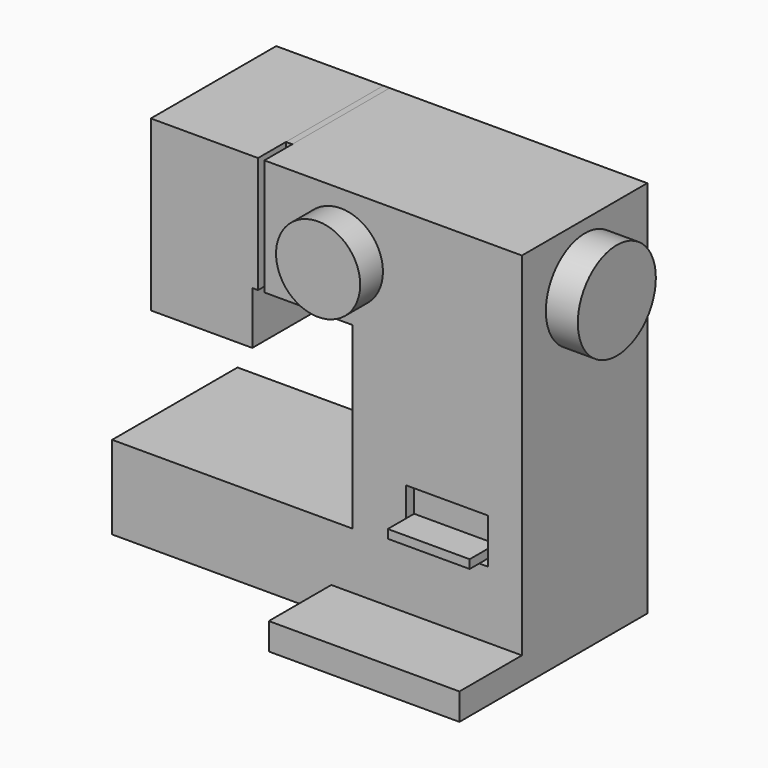
from build123d import *

# Parameters (mm, degrees)
F2_DEPTH = 76.2
F0_R     = 20.4653135308
F3_DEPTH = 90.03188
F0_W     = 39.8295894265
F0_H     = 14.2082143575
F0_H_2   = 3.4938193858
F4_DEPTH = 71.26206
F0_H_3   = 4.1925944388
F5_DEPTH = 87.27823
F0_W_2   = 92.7027892321
F0_H_4   = 13.0436122417
F6_DEPTH = 114.18662
F0_W_3   = 3.078199923
F0_H_5   = 56.5431583673
F7_DEPTH = 59.22076
F1_R     = 23.7210403161
F8_DEPTH = 122.76001


with BuildPart() as f2:
    # F0 (on Front) → F2 (new body)
    with BuildSketch(Plane.XZ):
        Polygon((-73.2527300715, 87.5874310732), (-73.2527300715, 5.3862300701), (-23.8952767104, 5.3862300701), (-23.8952767104, 31.0442727059), (-21.1126040667, 31.0442727059), (-21.1126040667, 87.5874310732), align=None)
    extrude(amount=F2_DEPTH)


with BuildPart() as f2b:
    # F0 (on Front) → F2, piece 2 (new body)
    with BuildSketch(Plane.XZ):
        Polygon((107.2141155601, 87.5874310732), (-18.0344041437, 87.5874310732), (-18.0344041437, 31.0442727059), (24.8745921999, 31.0442727059), (24.8745921999, -56.1147257686), (-92.0555666089, -56.1147257686), (-92.0555666089, -96.6535285115), (14.5113263279, -96.6535285115), (14.5113263279, -83.6099162698), (107.2141155601, -83.6099162698), align=None)
        Polygon((90.6766802073, -51.0009080172), (50.8470907807, -51.0009080172), (50.8470907807, -47.5070886314), (50.8470907807, -43.3144941926), (50.8470907807, -29.1062798351), (90.6766802073, -29.1062798351), (90.6766802073, -43.3144941926), (90.6766802073, -47.5070886314), align=None, mode=Mode.SUBTRACT)
        with Locations((19.1697571427, 58.7051510811)):
            Circle(F0_R, mode=Mode.SUBTRACT)
    extrude(amount=F2_DEPTH)

    # F0 (on Front) → F3 (join)
    with BuildSketch(Plane.XZ):
        with Locations((19.1697571427, 58.7051510811)):
            Circle(F0_R)
    extrude(amount=F3_DEPTH)

    # F0 (on Front) → F4 (join)
    with BuildSketch(Plane.XZ):
        with Locations((70.761885494, -36.2103870139)):
            Rectangle(F0_W, F0_H)
        with Locations((70.761885494, -49.2539983243)):
            Rectangle(F0_W, F0_H_2)
    extrude(amount=F4_DEPTH)

    # F0 (on Front) → F5 (join)
    with BuildSketch(Plane.XZ):
        with Locations((70.761885494, -45.410791412)):
            Rectangle(F0_W, F0_H_3)
    extrude(amount=F5_DEPTH)

    # F0 (on Front) → F6 (join)
    with BuildSketch(Plane.XZ):
        with Locations((60.862720944, -90.1317223907)):
            Rectangle(F0_W_2, F0_H_4)
    extrude(amount=F6_DEPTH)

    # F1 (on Right) → F8 (join)
    with BuildSketch(Plane.YZ):
        with Locations((-37.9360765219, 57.8596889973)):
            Circle(F1_R)
    extrude(amount=F8_DEPTH)


with BuildPart() as f7:
    # F0 (on Front) → F7 (new body)
    with BuildSketch(Plane.XZ):
        with Locations((-19.5735041052, 59.3158518896)):
            Rectangle(F0_W_3, F0_H_5)
    extrude(amount=F7_DEPTH)


solid = Compound([f2.part, f2b.part, f7.part])
